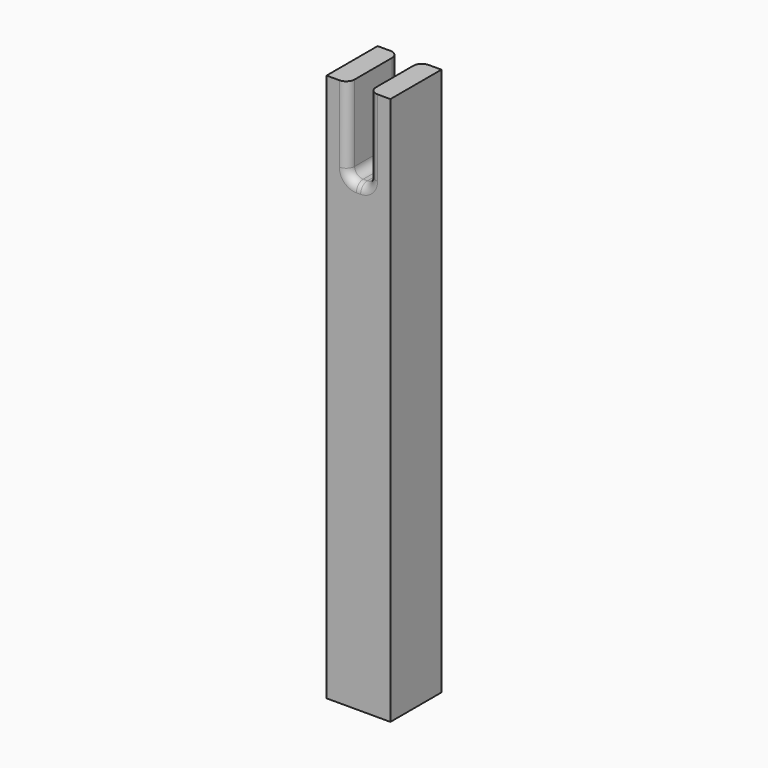
from build123d import *

# Parameters (mm, degrees)
F0_W     = 38.1
F0_H     = 38.1
F1_DEPTH = 327.5076
F2_W     = 12.7
F2_H     = 38.1
F3_DEPTH = 50.8
F4_F1_R  = 5.08
F4_F2_R  = 5.08


with BuildPart() as f1:
    # F0 (on Top) → F1 (new body)
    with BuildSketch(Plane.XY):
        with Locations((19.05, -19.05)):
            Rectangle(F0_W, F0_H)
    extrude(amount=F1_DEPTH)

    # F2 (on face) → F3 (cut)
    with BuildSketch(Plane.XY.offset(327.5076)):
        with Locations((19.05, -19.05)):
            Rectangle(F2_W, F2_H)
    extrude(amount=-F3_DEPTH, mode=Mode.SUBTRACT)

    # F4: fillet of radius 5.08 on 4 edges, made by hand

    # F4_f1
    f4_f1_edges = [f1.edges().sort_by_distance(p)[0] for p in [
        (12.7, -19.05, 276.7076),
        (25.4, -19.05, 276.7076),
    ]]
    fillet(f4_f1_edges, radius=F4_F1_R)

    # F4_f2
    f4_f2_edges = [f1.edges().sort_by_distance(p)[0] for p in [
        (19.05, 0, 276.7076),
        (19.05, -38.1, 276.7076),
        (14.1878975516, -38.1, 278.1954975516),
        (23.9121024484, -38.1, 278.1954975516),
        (23.9121024484, 0, 278.1954975516),
        (14.1878975516, 0, 278.1954975516),
    ]]
    fillet(f4_f2_edges, radius=F4_F2_R)


solid = f1.part
